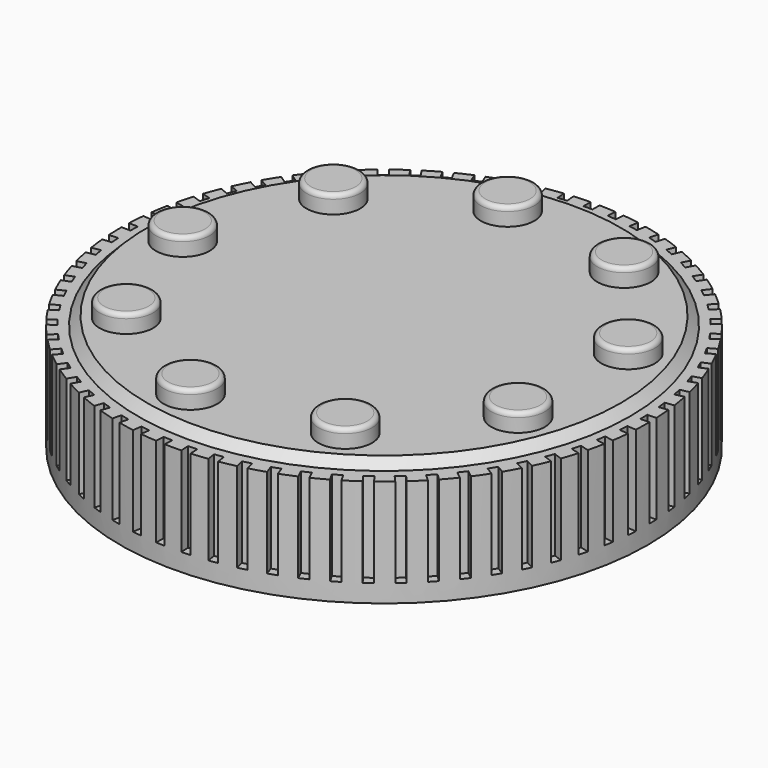
from build123d import *

# Parameters (mm, degrees)
F0_R            = 14.75
F1_DEPTH        = 6
F3_DEPTH        = 5
F3_COPIES_COUNT = 65
F4_R            = 13.75
F5_DEPTH        = 0.5
F7_DEPTH        = 1
F7_COPIES_COUNT = 9
F8_R            = 0.25
F9_SIZE         = 0.49999


# Not quite as in the source:
# - a fillet or chamfer is up to 0.001 mm smaller than in the source, because OpenCascade refuses the exact size
# - a pattern or mirror of a feature is missing from the dataset's text; its kind, count and spacing are read off the source's solid


with BuildPart() as f1:
    # F0 (on Top) → F1 (new body)
    with BuildSketch(Plane.XY):
        Circle(F0_R)
    extrude(amount=F1_DEPTH)

    # F2 (on face) → F3 (cut)
    with BuildSketch(Plane.XY.offset(6)):
        with BuildLine():
            ThreePointArc((0.25, 14.7478812038), (0, 14.75), (-0.25, 14.7478812038))
            Line((-0.25, 14.7478812038), (-0.25, 14.25))
            Line((-0.25, 14.25), (0.25, 14.25))
            Line((0.25, 14.25), (0.25, 14.7478812038))
        make_face()
    f3 = extrude(amount=-F3_DEPTH, mode=Mode.SUBTRACT)

    # F3_copies: F3 ×65 about axis
    f3_copies_axis = Axis((0, 0, 0), (0, 0, 1))
    for i in range(1, F3_COPIES_COUNT):
        add(f3.rotate(f3_copies_axis, i * 360 / F3_COPIES_COUNT), mode=Mode.SUBTRACT)

    # F4 (on face) → F5 (join)
    with BuildSketch(Plane.XY.offset(6)):
        Circle(F4_R)
    extrude(amount=F5_DEPTH)

    # F6 (on face) → F7 (join)
    with BuildSketch(Plane.XY.offset(6.5)):
        with BuildLine():
            ThreePointArc((-12.75, 0), (-11.25, -1.5), (-9.75, 0))
            ThreePointArc((-9.75, 0), (-11.25, 1.5), (-12.75, 0))
        make_face()
    f7 = extrude(amount=F7_DEPTH)

    # F7_copies: F7 ×9 about axis
    f7_copies_axis = Axis((0, 0, 0), (0, 0, 1))
    for i in range(1, F7_COPIES_COUNT):
        add(f7.rotate(f7_copies_axis, i * 360 / F7_COPIES_COUNT))

    # F8
    f8_edges = [f1.edges().sort_by_distance(p)[0] for p in [
        (-12.75, 0, 7.5),
        (-9.767067, -8.195542, 7.5),
        (-2.214014, -12.556299, 7.5),
        (6.375, -11.041824, 7.5),
        (11.981081, -4.360757, 7.5),
        (-9.767067, 8.195542, 7.5),
        (-2.214014, 12.556299, 7.5),
        (11.981081, 4.360757, 7.5),
        (6.375, 11.041824, 7.5),
    ]]
    fillet(f8_edges, radius=F8_R)

    # F9 (size 0.5 in the source; OpenCascade refuses exactly that, so slightly less here)
    f9_edges = [f1.edges().sort_by_distance(p)[0] for p in [
        (-13.75, 0, 6.5),
    ]]
    chamfer(f9_edges, length=F9_SIZE)


solid = f1.part
